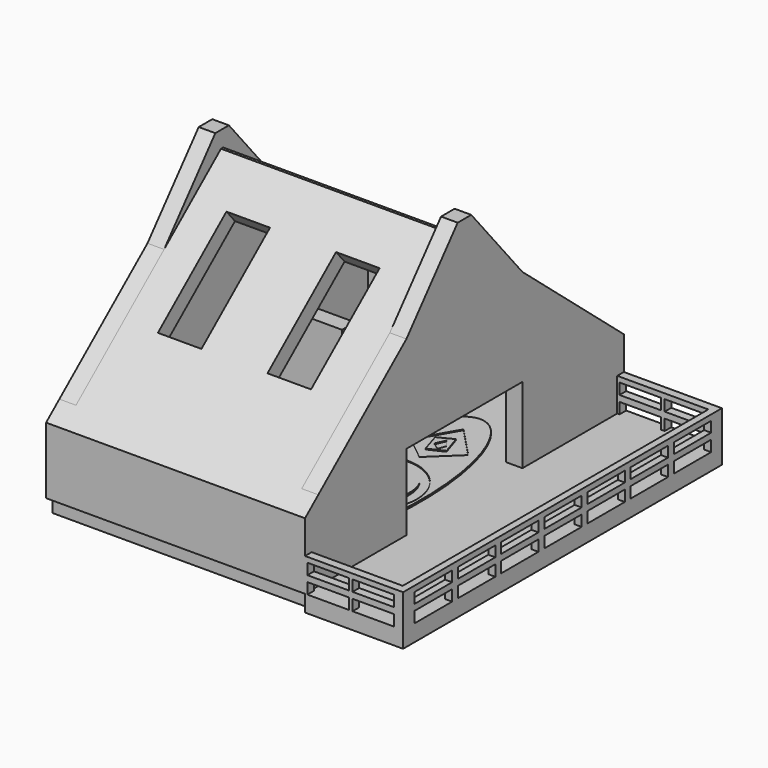
from build123d import *

# Parameters (mm, degrees)
F0_W         = 109.22
F0_H         = 121.92
F1_DEPTH     = 76.2
F2_W         = 29.999686
F2_H         = 121.92
F3_DEPTH     = 71.12
F4_C1_SIZE2  = 60.5410825038
F4_C1_SIZE   = 50.8
F4_C2_SIZE2  = 50.8
F4_C2_SIZE   = 60.5410825038
F5_T         = -5.08
F6_W         = 5.08
F6_H         = 111.76
F7_DEPTH     = 76.2
F8_T4_DEPTH  = 332.4105751248
F8_T9_DEPTH  = 332.4105751248
F8_T14_DEPTH = 332.4105751248
F6_W_2       = 27.8581011352
F6_H_2       = 2.54
F6_W_3       = 2.1415848648
F6_H_3       = 116.84
F11_DEPTH    = 10.16
F12_W        = 14.2918676138
F12_H        = 3.3658803758
F12_H_2      = 3.2075148208
F13_DEPTH    = 5.08
F14_W        = 12.7
F14_H        = 3.365881
F15_DEPTH    = 5.08
F16_W        = 12.7
F16_H        = 3.365881
F17_DEPTH    = 5.08
F18_W        = 44.3702784801
F18_H        = 23.2692971212
F19_DEPTH    = 5.08
F20_W        = 13.3246034384
F20_H        = 34.2183164025
F21_DEPTH    = 5.08
F6_W_4       = 2.8695403112
F6_H_4       = 38.9881794004
F6_W_5       = 23.1825265217
F6_H_5       = 4.9662292004
F22_DEPTH    = 22.86
F23_DEPTH    = 0.254
F24_R        = 14.1939412968
F25_DEPTH    = 0.254
F26_W        = 1.0243207216
F26_H        = 14.932422433
F27_DEPTH    = 2.54
F28_W        = 79.220314
F28_H        = 2.532
F28_H_2      = 2.913
F29_DEPTH    = 5.0546


# Not quite as in the source:
# - a fillet or chamfer that OpenCascade refuses, or shapes differently, is made with other operations: its cross-section is extruded or revolved along the edge and cut away or added
# - a feature of the source that left no trace in its solid (it failed there, or was rolled back) is left out
# - a feature names something its author has since deleted; it is built from what else it names


with BuildPart() as f1:
    # F0 (on Top) → F1 (new body)
    with BuildSketch(Plane.XY):
        with Locations((-15.1026358545, 32.3394851189)):
            Rectangle(F0_W, F0_H)
    extrude(amount=F1_DEPTH)

    # F2 (on face) → F3 (cut)
    with BuildSketch(Plane.XY.offset(76.2)):
        with Locations((24.5075211455, 32.3394851189)):
            Rectangle(F2_W, F2_H)
    extrude(amount=-F3_DEPTH, mode=Mode.SUBTRACT)

    # F4: chamfer of 50.8 x 60.5410825038 on 2 edges, made by hand

    # F4_c1
    f4_c1_edges = [f1.edges().sort_by_distance(p)[0] for p in [
        (-30.1024788545, 93.2994851189, 76.2),
    ]]
    f4_c1_side = f1.faces().sort_by_distance((-30.1024788545, 93.2994851189, 75.184))[0]
    chamfer(f4_c1_edges, length=F4_C1_SIZE, length2=F4_C1_SIZE2, reference=f4_c1_side)

    # F4_c2
    f4_c2_edges = [f1.edges().sort_by_distance(p)[0] for p in [
        (-30.1024788545, -28.6205148811, 76.2),
    ]]
    f4_c2_side = f1.faces().sort_by_distance((-30.1024788545, -27.6045148811, 76.2))[0]
    chamfer(f4_c2_edges, length=F4_C2_SIZE, length2=F4_C2_SIZE2, reference=f4_c2_side)

    # F5: a shell. OpenCascade refuses it in one call, so the cavity is built on its own and cut out:
    # the body offset inwards by the wall thickness, plus a prism from it out through each open face.
    f5_core = offset(f1.part, amount=F5_T, kind=Kind.INTERSECTION, mode=Mode.PRIVATE)
    f5_exits = [f5_core.faces().sort_by_distance(p)[0] for p in [
        (4.427678, 32.339485, 27.990765),
        (-64.632636, 32.339485, 27.990765),
    ]]
    add(f5_core, mode=Mode.SUBTRACT)
    extrude(f5_exits, amount=-F5_T, mode=Mode.SUBTRACT)

    # F6 (on face) → F7 (join)
    with BuildSketch(Plane.XY.offset(5.08)):
        Polygon((-69.7126358545, -23.5405148811), (-64.6326358545, -23.5405148811), (-64.6326358545, 49.2313057184), (-64.6326358545, 54.1975349188), (-64.6326358545, 88.2194851189), (-69.7126358545, 88.2194851189), align=None)
        with Locations((6.9676781455, 32.3394851189)):
            Rectangle(F6_W, F6_H)
    extrude(amount=F7_DEPTH)

    # F8: chamfer of 63.5 x 53.2828265798 on 3 edges, made by hand


with BuildPart() as f8_tool2:
    # F8_s3 → F8_t4 (new body)
    with BuildSketch(Plane.YZ.offset(173.1729657079)):
        Polygon((88.2194851189, 17.78), (34.9366585391, 81.28), (88.2194851189, 81.28), align=None)
    extrude(amount=-F8_T4_DEPTH)

    split(bisect_by=Plane(origin=(0, 51.0561582386, 60.8463600049), x_dir=(1, 0, 0), z_dir=(0, 0.6427876097, 0.7660444431)), keep=Keep.TOP)


with BuildPart() as f1_1:
    add(f1.part)

    # F8_t1: cut F8_tool2
    add(f8_tool2.part, mode=Mode.SUBTRACT)


with BuildPart() as f8_tool7:
    # F8_s8 → F8_t9 (new body)
    with BuildSketch(Plane.YZ.offset(99.0326517079)):
        Polygon((88.2194851189, 17.78), (34.9366585391, 81.28), (88.2194851189, 81.28), align=None)
    extrude(amount=-F8_T9_DEPTH)

    split(bisect_by=Plane(origin=(0, 51.0561582386, 60.8463600049), x_dir=(1, 0, 0), z_dir=(0, 0.6427876097, 0.7660444431)), keep=Keep.TOP)


with BuildPart() as f1_2:
    add(f1_1.part)

    # F8_t6: cut F8_tool7
    add(f8_tool7.part, mode=Mode.SUBTRACT)


with BuildPart() as f8_tool12:
    # F8_s13 → F8_t14 (new body)
    with BuildSketch(Plane.YZ.offset(-159.2376094169)):
        Polygon((29.7423116986, 81.28), (-23.5405148811, 17.78), (-23.5405148811, 81.28), align=None)
    extrude(amount=F8_T14_DEPTH)

    split(bisect_by=Plane(origin=(0, -24.3323657773, 28.9981843314), x_dir=(1, 0, 0), z_dir=(0, -0.6427876097, 0.7660444431)), keep=Keep.TOP)


with BuildPart() as f1_3:
    add(f1_2.part)

    # F8_t11: cut F8_tool12
    add(f8_tool12.part, mode=Mode.SUBTRACT)

    # F6 (on face) → F11 (join)
    with BuildSketch(Plane.XY.offset(5.08)):
        with Locations((23.4367287131, -27.3505148811)):
            Rectangle(F6_W_2, F6_H_2)
        with Locations((38.4365717131, -27.3505148811)):
            Rectangle(F6_W_3, F6_H_2)
        with Locations((38.4365717131, 32.3394851189)):
            Rectangle(F6_W_3, F6_H_3)
        with Locations((23.4367287131, 92.0294851189)):
            Rectangle(F6_W_2, F6_H_2)
        with Locations((38.4365717131, 92.0294851189)):
            Rectangle(F6_W_3, F6_H_2)
    extrude(amount=F11_DEPTH)

    # F12 (on face) → F13 (cut)
    with BuildSketch(Plane(origin=(37.3657792807, 0, 0), x_dir=(0, -1, 0), z_dir=(-1, 0, 0))):
        with Locations((-82.033649087, 6.7629402196)):
            Rectangle(F12_W, F12_H)
        with Locations((-82.033649087, 11.9161574421)):
            Rectangle(F12_W, F12_H_2)
        with Locations((-65.523649087, 6.7629402196)):
            Rectangle(F12_W, F12_H)
        with Locations((-65.523649087, 11.9161574421)):
            Rectangle(F12_W, F12_H_2)
        with Locations((-49.013649087, 6.7629402196)):
            Rectangle(F12_W, F12_H)
        with Locations((-49.013649087, 11.9161574421)):
            Rectangle(F12_W, F12_H_2)
        with Locations((-32.503649087, 6.7629402196)):
            Rectangle(F12_W, F12_H)
        with Locations((-32.503649087, 11.9161574421)):
            Rectangle(F12_W, F12_H_2)
        with Locations((-15.993649087, 6.7629402196)):
            Rectangle(F12_W, F12_H)
        with Locations((-15.993649087, 11.9161574421)):
            Rectangle(F12_W, F12_H_2)
        with Locations((0.516350913, 6.7629402196)):
            Rectangle(F12_W, F12_H)
        with Locations((0.516350913, 11.9161574421)):
            Rectangle(F12_W, F12_H_2)
        with Locations((17.026350913, 6.7629402196)):
            Rectangle(F12_W, F12_H)
        with Locations((17.026350913, 11.9161574421)):
            Rectangle(F12_W, F12_H_2)
    extrude(amount=-F13_DEPTH, mode=Mode.SUBTRACT)

    # F14 (on face) → F15 (cut)
    with BuildSketch(Plane(origin=(0, -26.0805148811, 0), x_dir=(-1, 0, 0), z_dir=(0, 1, 0))):
        with Locations((-30.3991394281, 6.7629405317)):
            Rectangle(F14_W, F14_H)
        with Locations((-30.3991394281, 11.9953405317)):
            Rectangle(F14_W, F14_H)
        with Locations((-16.5815394281, 6.7629405317)):
            Rectangle(F14_W, F14_H)
        with Locations((-16.5815394281, 11.9953405317)):
            Rectangle(F14_W, F14_H)
    extrude(amount=-F15_DEPTH, mode=Mode.SUBTRACT)

    # F16 (on face) → F17 (cut)
    with BuildSketch(Plane.XZ.offset(-90.7594851189)):
        with Locations((16.5621392265, 6.7629405317)):
            Rectangle(F16_W, F16_H)
        with Locations((16.5621392265, 11.9953405317)):
            Rectangle(F16_W, F16_H)
        with Locations((30.3797392265, 6.7629405317)):
            Rectangle(F16_W, F16_H)
        with Locations((30.3797392265, 11.9953405317)):
            Rectangle(F16_W, F16_H)
    extrude(amount=-F17_DEPTH, mode=Mode.SUBTRACT)

    # F18 (on face) → F19 (cut)
    with BuildSketch(Plane.YZ.offset(9.5076781455)):
        with Locations((32.3394851189, 16.7146485606)):
            Rectangle(F18_W, F18_H)
    extrude(amount=-F19_DEPTH, mode=Mode.SUBTRACT)

    # F20 (on face) → F21 (cut)
    with BuildSketch(Plane(origin=(0, -24.3323657773, 28.9981843314), x_dir=(1, 0, 0), z_dir=(0, -0.6427876097, 0.7660444431))):
        with Locations((-47.6010553539, 42.1169388426)):
            Rectangle(F20_W, F20_H)
        with Locations((-14.0730553539, 42.1169388426)):
            Rectangle(F20_W, F20_H)
    extrude(amount=-F21_DEPTH, mode=Mode.SUBTRACT)

    # F6 (on face) → F22 (join)
    with BuildSketch(Plane.XY.offset(5.08)):
        Polygon((-69.7126358545, -23.5405148811), (-64.6326358545, -23.5405148811), (-64.6326358545, 49.2313057184), (-64.6326358545, 54.1975349188), (-64.6326358545, 88.2194851189), (-69.7126358545, 88.2194851189), align=None)
        with Locations((-31.5372490101, 68.7253954186)):
            Rectangle(F6_W_4, F6_H_4)
        with Locations((-53.0413725937, 51.7144203186)):
            Rectangle(F6_W_5, F6_H_5)
    extrude(amount=F22_DEPTH)

    # F6 (on face) → F23 (join)
    with BuildSketch(Plane.XY.offset(5.08)):
        with BuildLine():
            add(Edge.make_bspline(
                [(-13.5902510956, 67.3234462738), (-39.5377666614, 67.3234462738), (-26.5640088785, 5.4330518469), (-13.5902510956, -56.45734258), (-0.6164933127, 5.4330518469), (12.3572644702, 67.3234462738), (-13.5902510956, 67.3234462738)],
                knots=[0, 0, 0, 2.0943951024, 2.0943951024, 4.1887902048, 4.1887902048, 6.2831853072, 6.2831853072, 6.2831853072], degree=2, weights=[1, 0.5, 1, 0.5, 1, 0.5, 1]))
        make_face()
    extrude(amount=F23_DEPTH)

    # F24 (on face) → F25 (join)
    with BuildSketch(Plane.XY.offset(5.334)):
        with BuildLine():
            add(Edge.make_bspline(
                [(-13.5902510956, 67.3234462738), (-39.5377666614, 67.3234462738), (-26.5640088785, 5.4330518469), (-13.5902510956, -56.45734258), (-0.6164933127, 5.4330518469), (12.3572644702, 67.3234462738), (-13.5902510956, 67.3234462738)],
                knots=[0, 0, 0, 2.0943951024, 2.0943951024, 4.1887902048, 4.1887902048, 6.2831853072, 6.2831853072, 6.2831853072], degree=2, weights=[1, 0.5, 1, 0.5, 1, 0.5, 1]))
        make_face()
        Polygon((-18.0212110281, -12.0888184756), (-23.3488995582, -0.9161885828), (-15.8006395568, 2.5068330816), (-15.5625507358, 2.9932858644), (-15.1390045963, 2.806874522), (-11.1945960186, 4.5956041117), (-5.9772475621, -6.3456329741), align=None, mode=Mode.SUBTRACT)
        with Locations((-13.755351305, 25.5152142818)):
            Circle(F24_R, mode=Mode.SUBTRACT)
        Polygon((-12.7351997185, 42.8974415477), (-20.2279090881, 48.9118620753), (-13.4408962012, 60.6738972515), (-4.2294830619, 50.9788706775), align=None, mode=Mode.SUBTRACT)
        with BuildLine():
            ThreePointArc((-19.0662875707, 26.3796935066), (-18.7179582892, 28.8257621837), (-17.3962920599, 30.913292696))
            ThreePointArc((-17.3962920599, 30.913292696), (-19.0756559721, 28.6257515073), (-19.4067303091, 25.8073303849))
            ThreePointArc((-19.4067303091, 25.8073303849), (-10.5397027926, 17.9244779909), (-2.6568503986, 26.7915055074))
            ThreePointArc((-2.6568503986, 26.7915055074), (-3.0929678811, 29.6485647533), (-4.2711682229, 32.2876611797))
            ThreePointArc((-4.2711682229, 32.2876611797), (-3.2624735175, 29.4374560196), (-3.0978869181, 26.4185082369))
            ThreePointArc((-3.0978869181, 26.4185082369), (-11.0677831154, 20.5143746158), (-19.0662875707, 26.3796935066))
        make_face()
        Polygon((-16.9349834323, 0.1891907305), (-16.8430920683, 0.3769391915), (-18.0729366839, 0.3769391915), (-18.0729366839, -6.7094038241), (-11.5555701777, -6.9163041189), (-11.5555701777, 0.3769391915), (-13.9473809482, 0.3769391915), (-14.3487267196, -0.5349605344), align=None)
        Polygon((-11.6567146396, 55.5984135734), (-16.2046384066, 53.3008873463), (-14.3593540415, 47.221768383), (-9.6690248281, 49.4583602501), align=None)
        Polygon((-12.0141894348, 48.9118620753), (-14.3593540415, 50.5943223834), (-12.9860220477, 53.6666363478), (-11.1864142251, 51.2883085934), align=None, mode=Mode.SUBTRACT)
        with BuildLine():
            ThreePointArc((-13.9204515144, 26.0631833225), (-13.755351305, 24.9429135316), (-13.5902510956, 26.0631833225))
            ThreePointArc((-13.5902510956, 26.0631833225), (-13.8318978291, 26.9541048328), (-14.6170496452, 26.4686453527))
            ThreePointArc((-14.6170496452, 26.4686453527), (-14.1372980762, 26.4917543954), (-13.9204515144, 26.0631833225))
        make_face()
    extrude(amount=F25_DEPTH)

    # F26 (on face) → F27 (join)
    with BuildSketch(Plane.XY.offset(5.08)):
        with Locations((-58.7432421744, -10.68279217)):
            Rectangle(F26_W, F26_H)
    extrude(amount=F27_DEPTH)

    # F28 (on face) → F29 (cut)
    with BuildSketch(Plane(origin=(0, 0, 0), x_dir=(1, 0, 0), z_dir=(0, 0, -1))):
        with Locations((-30.1024788545, 27.3545148811)):
            Rectangle(F28_W, F28_H)
        with Locations((-30.1024788545, -91.8429851189)):
            Rectangle(F28_W, F28_H_2)
    extrude(amount=-F29_DEPTH, mode=Mode.SUBTRACT)


solid = f1_3.part
